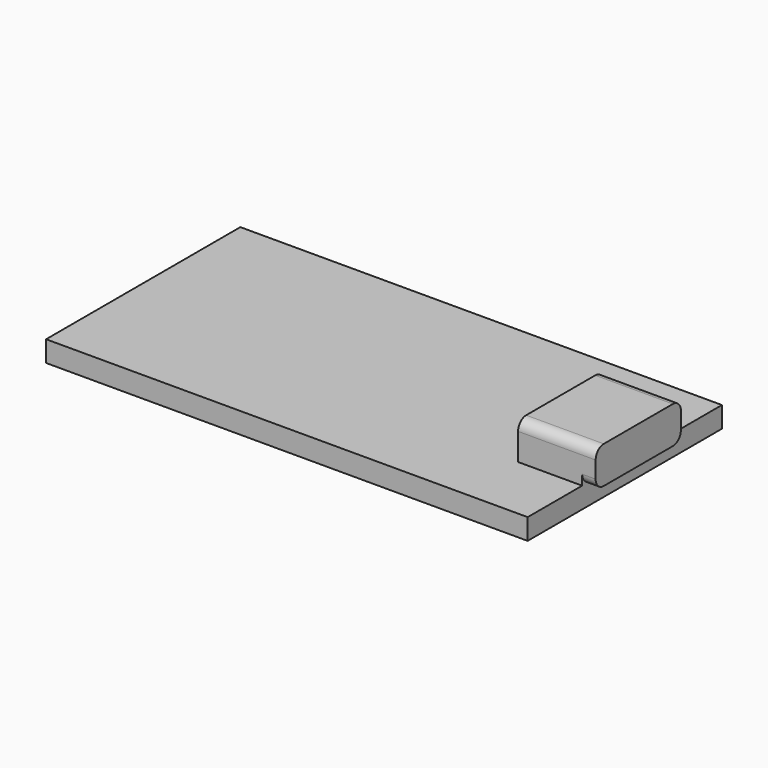
from build123d import *

# Parameters (mm, degrees)
F0_W     = 35.7
F0_H     = 18
F1_DEPTH = 1.55
F2_W     = 5.75
F2_H     = 7.9
F3_DEPTH = 2.75
F4_R     = 0.75


with BuildPart() as f1:
    # F0 (on Top) → F1 (new body)
    with BuildSketch(Plane.XY):
        Rectangle(F0_W, F0_H)
    extrude(amount=F1_DEPTH)

    # F2 (on face) → F3 (join)
    with BuildSketch(Plane.XY.offset(1.55)):
        with Locations((15.975, 0)):
            Rectangle(F2_W, F2_H)
    extrude(amount=F3_DEPTH)

    # F4
    f4_edges = [f1.edges().sort_by_distance(p)[0] for p in [
        (15.975, 3.95, 4.3),
        (15.975, -3.95, 4.3),
        (18.35, 3.95, 1.55),
        (18.35, -3.95, 1.55),
    ]]
    fillet(f4_edges, radius=F4_R)


solid = f1.part
